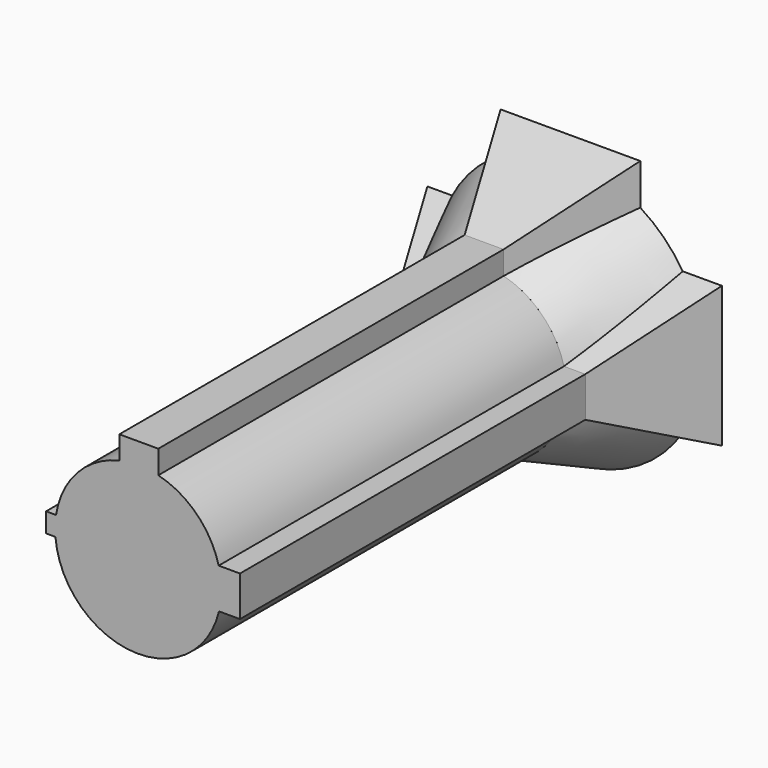
from build123d import *

# Parameters (mm, degrees)
F1_DEPTH               = 100
F2_DEPTH               = 25
DRAFT_F2_DRAFTED_ANGLE = -25


# Not quite as in the source:
# - an extrude with a draft is written as a straight extrude whose walls are then drafted


with BuildPart() as f1:
    # F0 (on Front) → F1 (new body)
    with BuildSketch(Plane.XZ):
        with BuildLine():
            ThreePointArc((18.2801916957, -11.4262133485), (18.6802080847, -9.1907481248), (18.8141683839, -6.9237297049))
            ThreePointArc((18.8141683839, -6.9237297049), (18.661709103, -4.5058249045), (18.2067462757, -2.1262206764))
            ThreePointArc((18.2067462757, -2.1262206764), (13.124788827, 6.7388303737), (4.2217151418, 11.7538777899))
            ThreePointArc((4.2217151418, 11.7538777899), (-0.2903711802, 12.3251515552), (-4.8105457618, 11.8218639198))
            ThreePointArc((-4.8105457618, 11.8218639198), (-14.5756539772, 6.1372667325), (-19.4686017558, -4.0475771877))
            ThreePointArc((-19.4686017558, -4.0475771877), (-19.6746472002, -6.3021743203), (-19.6145553546, -8.5653693904))
            ThreePointArc((-19.6145553546, -8.5653693904), (-1.8843598161, -26.1185343763), (18.2801916957, -11.4262133485))
        make_face()
        with BuildLine():
            ThreePointArc((-4.8105457618, 11.8218639198), (-0.2903711802, 12.3251515552), (4.2217151418, 11.7538777899))
            Line((4.2217151418, 11.7538777899), (4.2217151418, 11.8218639198))
            Line((4.2217151418, 11.8218639198), (4.2217151418, 17.1749683448))
            Line((4.2217151418, 17.1749683448), (-4.8105457618, 17.1749683448))
            Line((-4.8105457618, 17.1749683448), (-4.8105457618, 11.8218639198))
        make_face()
        with BuildLine():
            Line((-21.7770793319, -8.5653693904), (-19.6145553546, -8.5653693904))
            ThreePointArc((-19.6145553546, -8.5653693904), (-19.6746472002, -6.3021743203), (-19.4686017558, -4.0475771877))
            Line((-19.4686017558, -4.0475771877), (-19.6145553546, -4.0475771877))
            Line((-19.6145553546, -4.0475771877), (-21.7770793319, -4.0475771877))
            Line((-21.7770793319, -4.0475771877), (-21.7770793319, -8.5653693904))
        make_face()
        with BuildLine():
            ThreePointArc((18.2067462757, -2.1262206764), (18.661709103, -4.5058249045), (18.8141683839, -6.9237297049))
            ThreePointArc((18.8141683839, -6.9237297049), (18.6802080847, -9.1907481248), (18.2801916957, -11.4262133485))
            Line((18.2801916957, -11.4262133485), (23.1402359128, -11.4262133485))
            Line((23.1402359128, -11.4262133485), (23.1402359128, -2.1262206764))
            Line((23.1402359128, -2.1262206764), (18.2067462757, -2.1262206764))
        make_face()
    extrude(amount=F1_DEPTH)


with BuildPart() as f2_drafted:
    # F2 (new): a face of the model
    f2_faces = [f1.part.faces().sort_by_distance(p)[0] for p in [
        (0.1240427992, 0, -6.1363280025),
    ]]
    extrude(f2_faces, amount=F2_DEPTH)

    # draft_F2_drafted
    draft_f2_drafted_walls = [f2_drafted.faces().sort_by_distance(p)[0] for p in [
        (4.2217151418, 16.6666666667, 14.4644230674),
        (-0.29441531, 16.6666666667, 17.1749683448),
        (-4.8105457618, 16.6666666667, 14.4984161323),
        (-14.5756539772, 16.6666666667, 6.1372667325),
        (-20.6228405438, 16.6666666667, -4.0475771877),
        (-21.7770793319, 16.6666666667, -6.3064732891),
        (-20.6958173432, 16.6666666667, -8.5653693904),
        (-1.8843598161, 16.6666666667, -26.1185343763),
        (20.7102138042, 16.6666666667, -11.4262133485),
        (23.1402359128, 16.6666666667, -6.7762170124),
        (20.6734910943, 16.6666666667, -2.1262206764),
        (13.124788827, 16.6666666667, 6.7388303737),
    ]]
    draft(draft_f2_drafted_walls, neutral_plane=Plane(origin=(0.1240427992, 0, -6.1363280025), x_dir=(1, 0, 0), z_dir=(0, 1, 0)), angle=DRAFT_F2_DRAFTED_ANGLE)


with BuildPart() as f1_1:
    add(f1.part)

    # join_F2_drafted: union F2_drafted
    add(f2_drafted.part)


solid = f1_1.part
